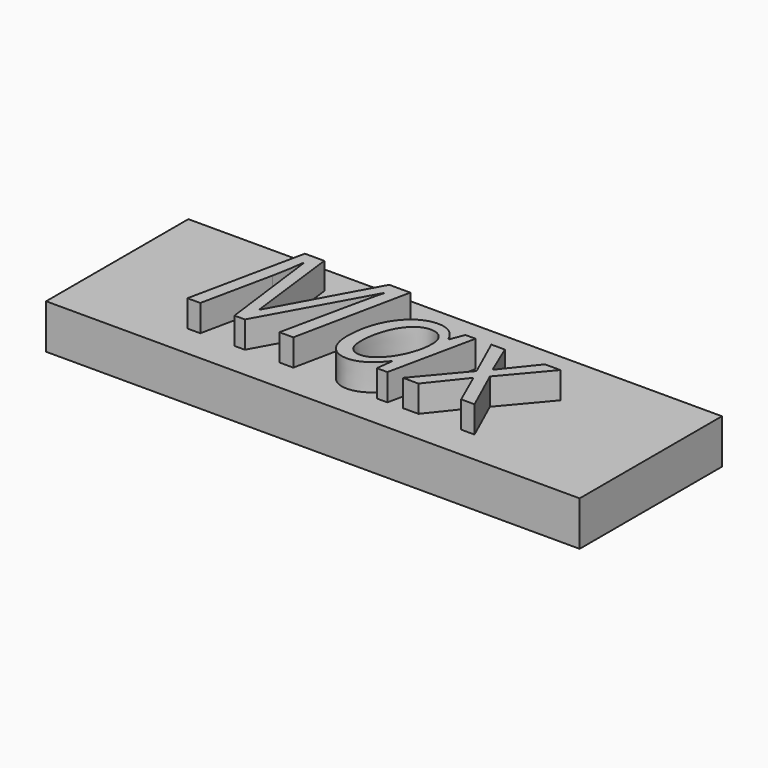
from build123d import *

# Parameters (mm, degrees)
F0_W         = 60
F0_H         = 20
F1_DEPTH     = 5
F2_TEXT_SIZE = 18.2964334575
F3_DEPTH     = 3


# Not quite as in the source:
# - Text() gives the source's letters only with a copy of the font that has no kerning and outlines rounded to 1/6400 em; it was checked with that copy


with BuildPart() as f1:
    # F0 (on Top) → F1 (new body)
    with BuildSketch(Plane.XY):
        Rectangle(F0_W, F0_H)
    extrude(amount=F1_DEPTH)

    # F2 (on face) → F3 (join)
    with BuildSketch(Plane.XY.offset(5)):
        with Locations((-17.8228798322, -6.2961252406)):
            Text('Max', F2_TEXT_SIZE, font='Open Sans', font_style=FontStyle.ITALIC, text_align=(TextAlign.LEFT, TextAlign.BOTTOM))
    extrude(amount=F3_DEPTH)


solid = f1.part
